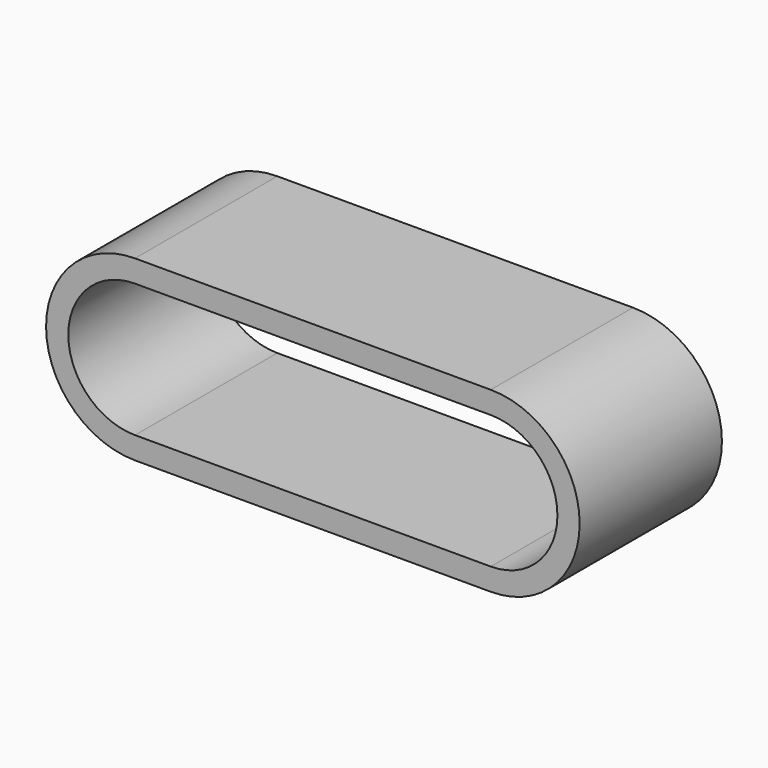
from build123d import *

# Parameters (mm, degrees)
F2_DEPTH      = 200
F2_DEPTH_BACK = 200
F4_DEPTH      = 4000


with BuildPart() as f2:
    # F1 (on face) → F2 (new body, two sides)
    with BuildSketch(Plane.XZ) as f2_sk:
        with BuildLine():
            Line((-400, -200), (400, -200))
            ThreePointArc((400, -200), (600, 0), (400, 200))
            Line((400, 200), (-400, 200))
            ThreePointArc((-400, 200), (-600, 0), (-400, -200))
        make_face()
    extrude(amount=-F2_DEPTH)
    extrude(f2_sk.sketch, amount=F2_DEPTH_BACK)

    # F3 (on face) → F4 (cut)
    with BuildSketch(Plane.XZ.offset(200)):
        with BuildLine():
            Line((-400, -150), (400, -150))
            ThreePointArc((400, -150), (550, 0), (400, 150))
            Line((400, 150), (-400, 150))
            ThreePointArc((-400, 150), (-550, 0), (-400, -150))
        make_face()
    extrude(amount=-F4_DEPTH, mode=Mode.SUBTRACT)


solid = f2.part
